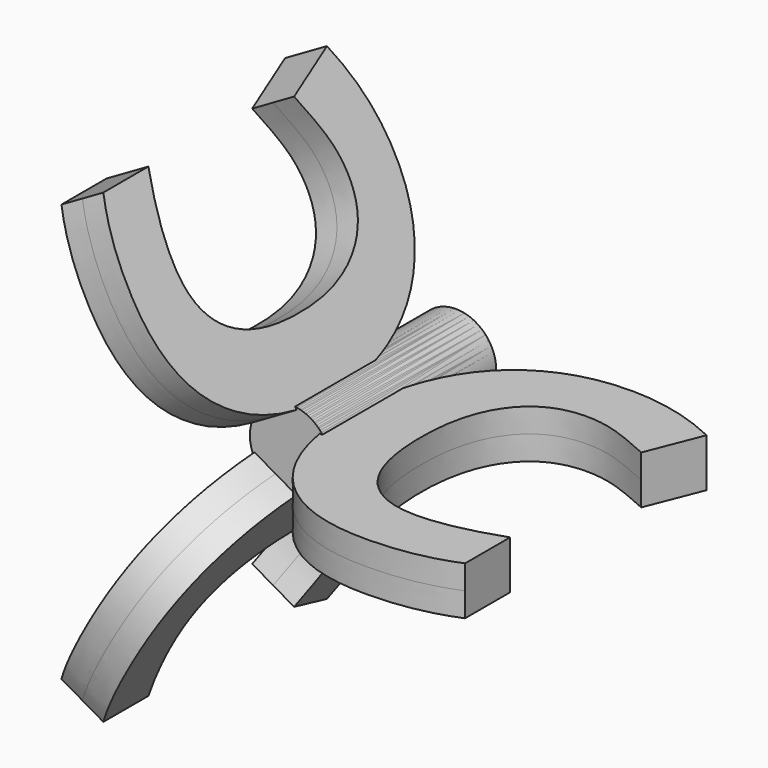
from build123d import *

# Parameters (mm, degrees)
F0_TEXT_SIZE = 45.8338014055
F1_DEPTH     = 2.5
F2_R         = 4.1650370023
F3_DEPTH     = 21.4
F4_COUNT     = 3


# Not quite as in the source:
# - Text() gives the source's letters only with a copy of the font that has no kerning and outlines rounded to 1/6400 em; it was checked with that copy


with BuildPart() as f1:
    # F0 (on Top) → F1 (new body, symmetric)
    with BuildSketch(Plane.XY):
        with Locations((0, -33.0003370119)):
            Text('C', F0_TEXT_SIZE, font='Open Sans', font_style=FontStyle.BOLD, text_align=(TextAlign.LEFT, TextAlign.BOTTOM))
    extrude(amount=F1_DEPTH, both=True)

    # F2 (on Front) → F3 (join)
    with BuildSketch(Plane.XZ):
        Circle(F2_R)
    extrude(amount=F3_DEPTH)


with BuildPart() as f4_1:
    # F4: instance of F1
    add(f1.part.rotate(Axis((0, 0, 0), (0, 1, 0)), 1 * 360 / F4_COUNT))


with BuildPart() as f4_2:
    # F4: instance of F1
    add(f1.part.rotate(Axis((0, 0, 0), (0, 1, 0)), 2 * 360 / F4_COUNT))


solid = Compound([f1.part, f4_1.part, f4_2.part])
